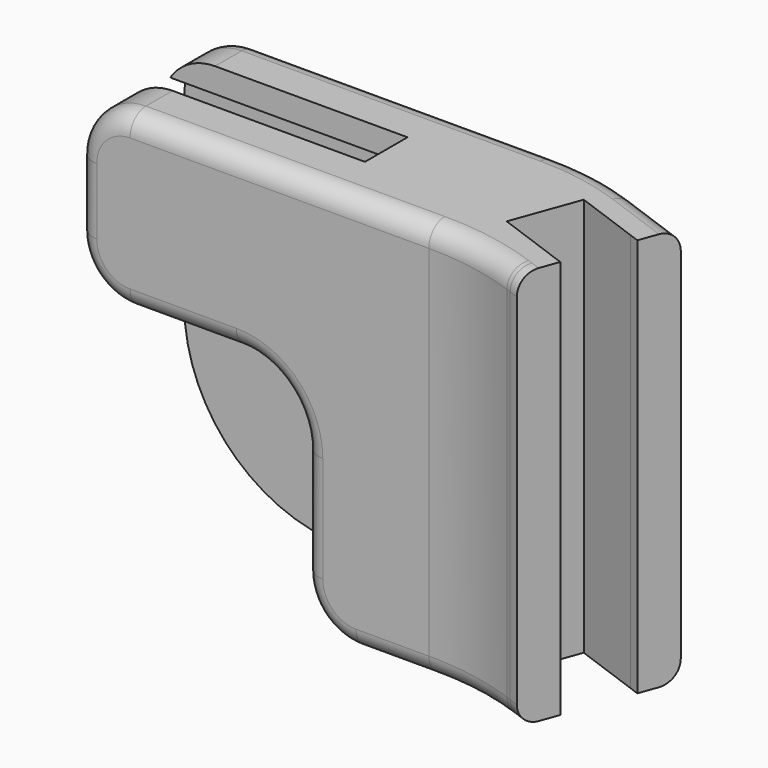
from build123d import *

# Parameters (mm, degrees)
F0_W         = 30
F0_H         = 12
F1_DEPTH     = 30
F2_W         = 8.215
F2_H         = 28.15
F3_DEPTH     = 28
F4_W         = 5.3
F4_H         = 30
F5_DEPTH     = 5.3
F6_W         = 17
F6_H         = 17
F7_DEPTH     = 2.8
F8_DEPTH     = 0.75
F9_R         = 12
F10_T1_DEPTH = 32
F10_T3_DEPTH = 11.8925
F11_R        = 20
F12_R        = 5
F13_R        = 1.5
F14_R        = 2
F15_W        = 5.0863461345
F15_H        = 4
F15_W_2      = 14.4734603858
F16_DEPTH    = 30.0010001


# Not quite as in the source:
# - a fillet or chamfer that OpenCascade refuses, or shapes differently, is made with other operations: its cross-section is extruded or revolved along the edge and cut away or added


with BuildPart() as f1:
    # F0 (on Top) → F1 (new body)
    with BuildSketch(Plane.XY):
        with Locations((-15, 6)):
            Rectangle(F0_W, F0_H)
        Polygon((0, 12), (0, 0), (3.6608153082, -1.3324278053), (7.5175409663, 9.2638388534), align=None)
    extrude(amount=F1_DEPTH)

    # F2 (on face) → F3 (cut)
    with BuildSketch(Plane(origin=(-30, 0, 0), x_dir=(0, -1, 0), z_dir=(-1, 0, 0))):
        with Locations((-6, 14.075)):
            Rectangle(F2_W, F2_H)
    extrude(amount=-F3_DEPTH, mode=Mode.SUBTRACT)

    # F4 (on face) → F5 (cut)
    with BuildSketch(Plane(origin=(3.6608153082, -1.3324278053, 0), x_dir=(0.3420201433, 0.9396926208, 0), z_dir=(0.9396926208, -0.3420201433, 0))):
        with Locations((5.6381557247, 15)):
            Rectangle(F4_W, F4_H)
    extrude(amount=-F5_DEPTH, mode=Mode.SUBTRACT)

    # F6 (on face) → F7 (cut)
    with BuildSketch(Plane.XZ):
        with Locations((-21.5, 8.5)):
            Rectangle(F6_W, F6_H)
    extrude(amount=-F7_DEPTH, mode=Mode.SUBTRACT)

    # F8 (add): faces of the model
    f8_faces = [f1.faces().sort_by_distance(p)[0] for p in [
        (7.0065362417, 7.8598649113, 15),
        (4.1718200328, 0.0715461368, 15),
    ]]
    extrude(f8_faces, amount=F8_DEPTH)

    # F9
    f9_edges = [f1.edges().sort_by_distance(p)[0] for p in [
        (-30, 11.05375, 0),
    ]]
    fillet(f9_edges, radius=F9_R)

    # F10: fillet of radius 4 on 3 edges, made by hand

    # F10_s2 → F10_t1 (cut)
    with BuildSketch(Plane.XZ.offset(-22)):
        with BuildLine():
            ThreePointArc((-30, 26), (-28.8284271247, 28.8284271247), (-26, 30))
            Line((-26, 30), (-30, 30))
            Line((-30, 30), (-30, 26))
        make_face()
    extrude(amount=F10_T1_DEPTH, mode=Mode.SUBTRACT)

    # F10_s4 → F10_t3 (cut)
    with BuildSketch(Plane.XZ.offset(-1.8925)):
        with BuildLine():
            ThreePointArc((-30, 21), (-28.8284271247, 18.1715728753), (-26, 17))
            Line((-26, 17), (-30, 17))
            Line((-30, 17), (-30, 21))
        make_face()
        with BuildLine():
            ThreePointArc((-9, 0), (-11.8284271247, 1.1715728753), (-13, 4))
            Line((-13, 4), (-13, 0))
            Line((-13, 0), (-9, 0))
        make_face()
    extrude(amount=F10_T3_DEPTH, mode=Mode.SUBTRACT)

    # F11
    f11_edges = [f1.edges().sort_by_distance(p)[0] for p in [
        (0, 12, 15),
        (0, 0, 15),
    ]]
    fillet(f11_edges, radius=F11_R)

    # F12
    f12_edges = [f1.edges().sort_by_distance(p)[0] for p in [
        (-13, 0.94625, 17),
    ]]
    fillet(f12_edges, radius=F12_R)

    # F13
    f13_edges = [f1.edges().sort_by_distance(p)[0] for p in [
        (-14.464466, 0, 15.535534),
        (-22, 0, 17),
        (-28.828427, 0, 28.828427),
        (-14.76327, 0, 30),
        (-0.053576, -0.303845, 30),
        (3.839724, -1.397545, 30),
        (3.839724, -1.397545, 0),
        (-0.053576, -0.303845, 0),
        (-6.26327, 0, 0),
        (-11.828427, 0, 1.171573),
        (-13, 0, 8),
        (-14.76327, 12, 30),
        (-0.053576, 11.696155, 30),
        (-28.828427, 0, 18.171573),
        (-30, 0, 23.5),
        (-10.76327, 12, 0),
        (-0.053576, 11.696155, 0),
        (5.768087, 9.900588, 0),
        (5.768087, 9.900588, 30),
        (-28.828427, 12, 28.828427),
        (-30, 12, 19),
        (-26.485281, 12, 3.514719),
    ]]
    fillet(f13_edges, radius=F13_R)

    # F14
    f14_edges = [f1.edges().sort_by_distance(p)[0] for p in [
        (-2, 6, 28.15),
    ]]
    fillet(f14_edges, radius=F14_R)

    # F15 (on face) → F16 (cut, through all)
    with BuildSketch(Plane.XY.offset(30)):
        with Locations((-28.5431730673, 6)):
            Rectangle(F15_W, F15_H)
        with Locations((-18.7632698071, 6)):
            Rectangle(F15_W_2, F15_H)
    extrude(amount=-F16_DEPTH, mode=Mode.SUBTRACT)


solid = f1.part
